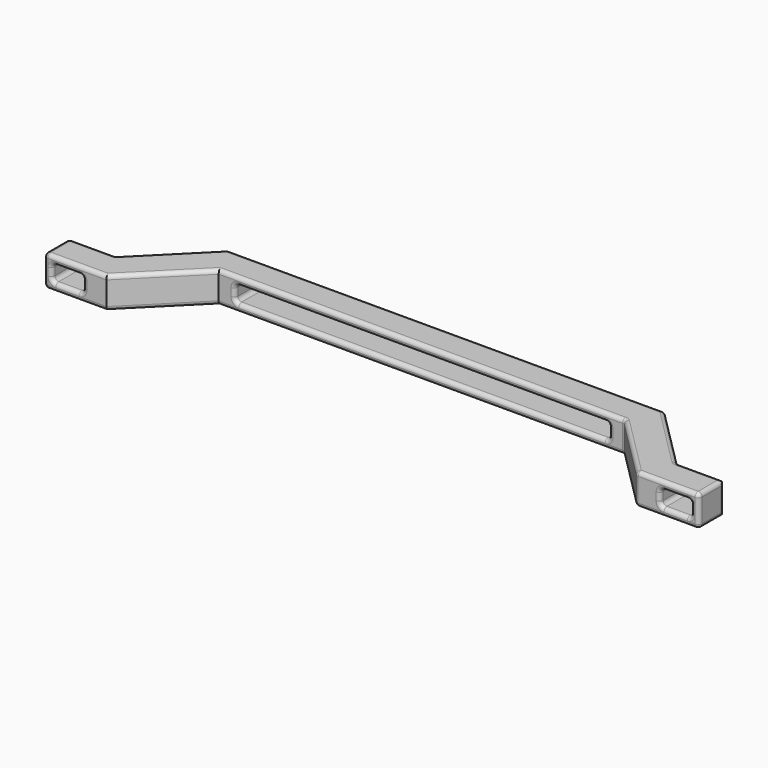
from build123d import *

# Parameters (mm, degrees)
F1_DEPTH    = 12.7
F2_W        = 152.4
F2_H        = 6.35
F3_DEPTH    = 45.1653850895
F4_F1_R     = 1.5875
F4_F2_R     = 1.5875
F5_W        = 12.7
F5_H        = 6.35
F6_DEPTH    = 38.101
F7_F1_R     = 1.5875
F7_F2_R     = 1.5875
F8_R        = 1.58749
F9_T1_DEPTH = 17.46252


# Not quite as in the source:
# - a fillet or chamfer that OpenCascade refuses, or shapes differently, is made with other operations: its cross-section is extruded or revolved along the edge and cut away or added
# - a fillet or chamfer is up to 0.001 mm smaller than in the source, because OpenCascade refuses the exact size


with BuildPart() as f1:
    # F0 (on Top) → F1 (new body)
    with BuildSketch(Plane.XY):
        Polygon((95.495135763, 45.1643850895), (-82.304864237, 45.1643850895), (-107.704864237, 19.7643850895), (-126.754864237, 19.7643850895), (-126.754864237, 7.0643850895), (-101.354864237, 7.0643850895), (-75.954864237, 32.4643850895), (89.145135763, 32.4643850895), (114.545135763, 7.0643850895), (139.945135763, 7.0643850895), (139.945135763, 19.7643850895), (120.895135763, 19.7643850895), align=None)
    extrude(amount=F1_DEPTH)

    # F2 (on Front) → F3 (cut, through all)
    with BuildSketch(Plane.XZ):
        with Locations((6.8134479225, 6.35)):
            Rectangle(F2_W, F2_H)
    extrude(amount=-F3_DEPTH, mode=Mode.SUBTRACT)

    # F4: fillet of radius 1.5875 on 6 edges, made by hand

    # F4_f1
    f4_f1_edges = [f1.edges().sort_by_distance(p)[0] for p in [
        (-69.3865520775, 38.8143850895, 3.175),
        (-69.3865520775, 38.8143850895, 9.525),
        (83.0134479225, 38.8143850895, 3.175),
        (83.0134479225, 38.8143850895, 9.525),
    ]]
    fillet(f4_f1_edges, radius=F4_F1_R)

    # F4_f2
    f4_f2_edges = [f1.edges().sort_by_distance(p)[0] for p in [
        (6.8134479225, 32.4643850895, 3.175),
        (6.8134479225, 45.1643850895, 3.175),
        (-68.9215840927, 45.1643850895, 3.6399679849),
        (82.5484799376, 45.1643850895, 3.6399679849),
        (82.5484799376, 32.4643850895, 3.6399679849),
        (-68.9215840927, 32.4643850895, 3.6399679849),
    ]]
    fillet(f4_f2_edges, radius=F4_F2_R)

    # F5 (on face) → F6 (cut, through all)
    with BuildSketch(Plane.XZ.offset(-7.0643850895)):
        with Locations((-117.229864237, 6.3499999233)):
            Rectangle(F5_W, F5_H)
        with Locations((130.420135763, 6.3499999233)):
            Rectangle(F5_W, F5_H)
    extrude(amount=-F6_DEPTH, mode=Mode.SUBTRACT)

    # F7: fillet of radius 1.5875 on 12 edges, made by hand

    # F7_f1
    f7_f1_edges = [f1.edges().sort_by_distance(p)[0] for p in [
        (-123.579864237, 13.4143850895, 9.5249999233),
        (-123.579864237, 13.4143850895, 3.1749999233),
        (-110.879864237, 13.4143850895, 3.1749999233),
        (-110.879864237, 13.4143850895, 9.5249999233),
        (124.070135763, 13.4143850895, 3.1749999233),
        (124.070135763, 13.4143850895, 9.5249999233),
        (136.770135763, 13.4143850895, 9.5249999233),
        (136.770135763, 13.4143850895, 3.1749999233),
    ]]
    fillet(f7_f1_edges, radius=F7_F1_R)

    # F7_f2
    f7_f2_edges = [f1.edges().sort_by_distance(p)[0] for p in [
        (-117.229864237, 7.0643850895, 3.1749999233),
        (130.420135763, 7.0643850895, 3.1749999233),
        (-110.879864237, 19.7643850895, 6.3499999233),
        (124.070135763, 19.7643850895, 6.3499999233),
        (124.5351037479, 19.7643850895, 9.0600319384),
        (124.5351037479, 19.7643850895, 3.6399679081),
        (-111.3448322218, 19.7643850895, 3.6399679081),
        (-111.3448322218, 19.7643850895, 9.0600319384),
        (124.5351037479, 7.0643850895, 3.6399679081),
        (136.3051677782, 7.0643850895, 3.6399679081),
        (-123.1148962521, 7.0643850895, 3.6399679081),
        (-111.3448322218, 7.0643850895, 3.6399679081),
    ]]
    fillet(f7_f2_edges, radius=F7_F2_R)

    # F8 (radius 1.5875 in the source; OpenCascade refuses exactly that, so slightly less here)
    f8_edges = [f1.edges().sort_by_distance(p)[0] for p in [
        (6.595136, 45.164385, 12.7),
        (6.595136, 45.164385, 0),
        (-95.004864, 32.464385, 12.7),
        (-82.304864, 45.164385, 6.35),
        (-107.704864, 19.764385, 6.35),
        (-95.004864, 32.464385, 0),
        (120.895136, 19.764385, 6.35),
        (95.495136, 45.164385, 6.35),
        (108.195136, 32.464385, 0),
        (108.195136, 32.464385, 12.7),
        (-117.229864, 19.764385, 12.7),
        (-126.754864, 13.414385, 12.7),
        (-114.054864, 7.064385, 12.7),
        (-88.654864, 19.764385, 12.7),
        (6.595136, 32.464385, 12.7),
        (101.845136, 19.764385, 12.7),
        (127.245136, 7.064385, 12.7),
        (139.945136, 13.414385, 12.7),
        (130.420136, 19.764385, 12.7),
        (-117.229864, 19.764385, 0),
        (-126.754864, 13.414385, 0),
        (-114.054864, 7.064385, 0),
        (-88.654864, 19.764385, 0),
        (6.595136, 32.464385, 0),
        (101.845136, 19.764385, 0),
        (127.245136, 7.064385, 0),
        (139.945136, 13.414385, 0),
        (130.420136, 19.764385, 0),
        (130.420136, 7.064385, 1.5875),
        (123.412572, 7.064385, 2.517436),
        (137.4277, 7.064385, 2.517436),
        (122.482636, 7.064385, 6.35),
        (138.357636, 7.064385, 6.35),
        (123.412572, 7.064385, 10.182564),
        (137.4277, 7.064385, 10.182564),
        (130.420136, 7.064385, 11.1125),
        (114.545136, 7.064385, 6.35),
        (139.945136, 7.064385, 6.35),
        (89.145136, 32.464385, 6.35),
        (-126.754864, 19.764385, 6.35),
        (-126.754864, 7.064385, 6.35),
    ]]
    fillet(f8_edges, radius=F8_R)

    # F9: fillet of radius 1.5875 on 4 edges, made by hand

    # F9_s2 → F9_t1 (cut)
    with BuildSketch(Plane.XY.offset(-2.38126)):
        with BuildLine():
            ThreePointArc((138.357635763, 19.7643850895), (139.4801677782, 19.2994171047), (139.945135763, 18.1768850895))
            Line((139.945135763, 18.1768850895), (139.945135763, 19.7643850895))
            Line((139.945135763, 19.7643850895), (138.357635763, 19.7643850895))
        make_face()
    extrude(amount=F9_T1_DEPTH, mode=Mode.SUBTRACT)


solid = f1.part
